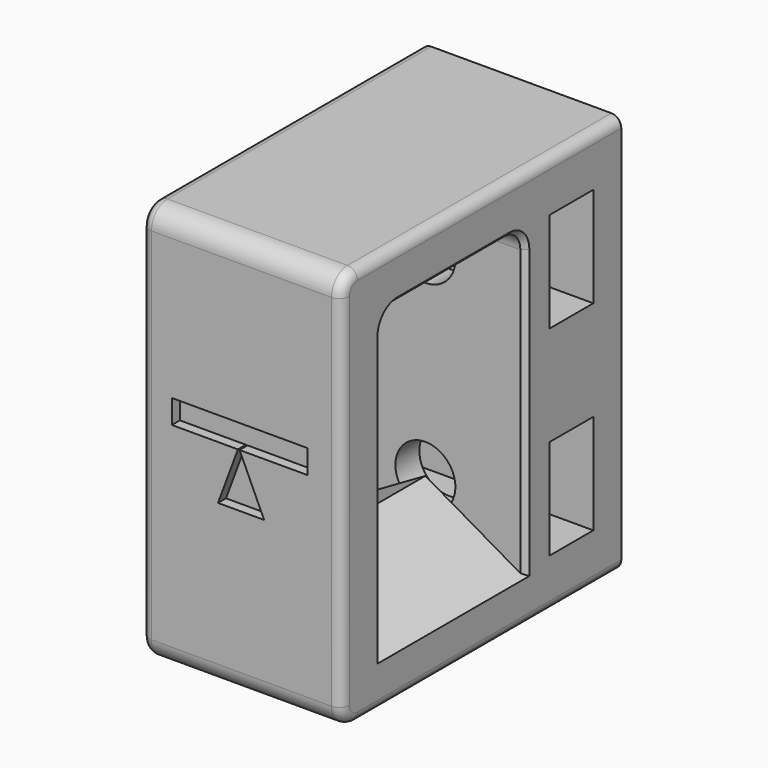
from build123d import *

# Parameters (mm, degrees)
F0_W      = 20
F0_H      = 40
F1_DEPTH  = 12
F2_R      = 3
F3_DEPTH  = 12
F5_DEPTH  = 23
F7_DEPTH  = 20
F8_R      = 1.99999
F9_R      = 1
F10_W     = 5.5
F10_H     = 10
F11_DEPTH = 25
F13_DEPTH = 1
F14_SIZE  = 0.5


# Not quite as in the source:
# - a fillet or chamfer is up to 0.001 mm smaller than in the source, because OpenCascade refuses the exact size


with BuildPart() as f1:
    # F0 (on Front) → F1 (new body)
    with BuildSketch(Plane.XZ):
        with Locations((10, 20)):
            Rectangle(F0_W, F0_H)
    extrude(amount=F1_DEPTH)

    # F2 (on face) → F3 (cut, through all)
    with BuildSketch(Plane(origin=(0, 0, 0), x_dir=(-1, 0, 0), z_dir=(0, 1, 0))):
        with Locations((-10, 30)):
            Circle(F2_R)
        with Locations((-10, 10)):
            Circle(F2_R)
    extrude(amount=-F3_DEPTH, mode=Mode.SUBTRACT)

    # F4 (on face) → F5 (join)
    with BuildSketch(Plane.XZ.offset(12)):
        Polygon((0, 4.2264973081), (0, 0), (20, 0), (20, 4.2264973081), (10, 10), align=None)
    extrude(amount=F5_DEPTH)

    # F6 (on face) → F7 (join, through all)
    with BuildSketch(Plane.YZ.offset(20)):
        Polygon((-35, 40), (-35, 4.2264973081), (-30, 4.2264973081), (-30, 35), (-12, 35), (-12, 40), align=None)
    extrude(amount=-F7_DEPTH)

    # F8 (radius 2 in the source; OpenCascade refuses exactly that, so slightly less here)
    f8_edges = [f1.edges().sort_by_distance(p)[0] for p in [
        (10, -35, 40),
        (10, -35, 0),
        (10, -30, 35),
        (10, -12, 35),
    ]]
    fillet(f8_edges, radius=F8_R)

    # F9
    f9_edges = [f1.edges().sort_by_distance(p)[0] for p in [
        (20, -35, 20),
        (0, -35, 20),
    ]]
    fillet(f9_edges, radius=F9_R)

    # F10 (on face) → F11 (cut)
    with BuildSketch(Plane.YZ.offset(20)):
        with Locations((-6.25, 30)):
            Rectangle(F10_W, F10_H)
        with Locations((-6.25, 10)):
            Rectangle(F10_W, F10_H)
    extrude(amount=-F11_DEPTH, mode=Mode.SUBTRACT)

    # F12 (on face) → F13 (cut)
    with BuildSketch(Plane.XZ.offset(35)):
        Polygon((16.5859262925, 23.9497199655), (3.0391060282, 23.9497199655), (3.0391060282, 21.5699486434), (9.6455384046, 21.5699486434), (9.8125161603, 21.5699486434), (16.5859262925, 21.5699486434), align=None)
        Polygon((9.8125161603, 21.5699486434), (9.6455384046, 21.5699486434), (7.6536308043, 16.2067040801), (12.2681558132, 16.2067040801), align=None)
    extrude(amount=-F13_DEPTH, mode=Mode.SUBTRACT)

    # F14
    f14_edges = [f1.edges().sort_by_distance(p)[0] for p in [
        (20, -12, 18.613254),
        (0, -12, 18.613254),
    ]]
    chamfer(f14_edges, length=F14_SIZE)


solid = f1.part
